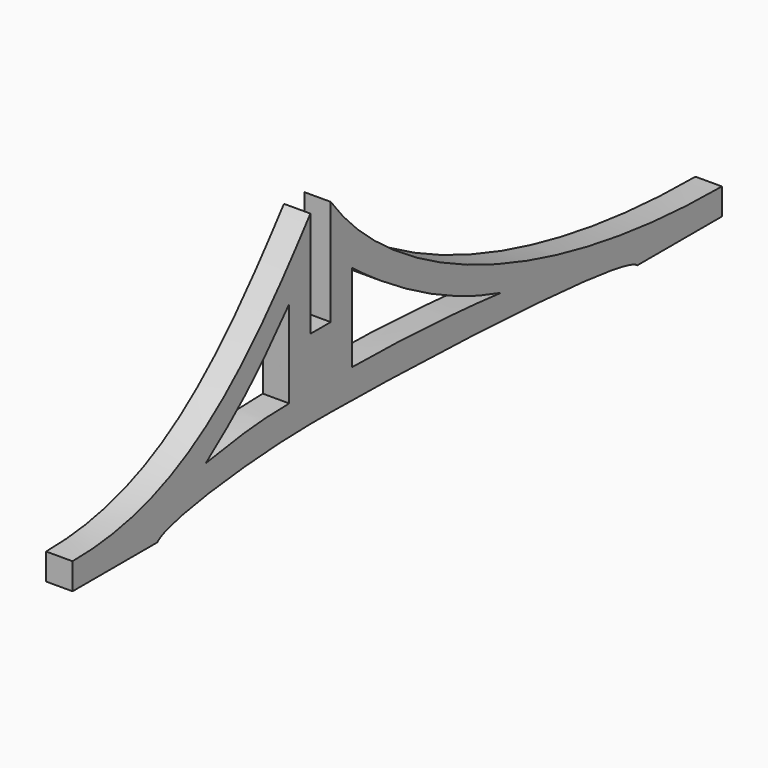
from build123d import *

# Parameters (mm, degrees)
F0_W     = 2.4
F0_H     = 15
F1_DEPTH = 5


# Not quite as in the source:
# - a feature names something its author has since deleted; it is built from what else it names


with BuildPart() as f1:
    # F0 (on Right) → F1 (new body)
    with BuildSketch(Plane.YZ):
        with Locations((-1.2, 12.5)):
            Rectangle(F0_W, F0_H)
        with Locations((1.2, 12.5)):
            Rectangle(F0_W, F0_H)
        with BuildLine():
            Line((2.4, 20), (2.4, 5))
            add(Edge.make_bspline(
                [(74.7971267972, 0), (71.3879865607, 3.4156564958), (16.494217181, 5), (2.4, 5)],
                knots=[0, 0, 0, 0, 72.5695801868, 72.5695801868, 72.5695801868, 72.5695801868], degree=3))
            Line((74.7971267972, 0), (94.7971267972, 0))
            Line((94.7971267972, 0), (94.7971267972, 5))
            add(Edge.make_bspline(
                [(2.4, 40), (16.6215170175, 20.5895993859), (51.1409416795, 5), (94.7971267972, 5)],
                knots=[0, 0, 0, 0, 98.8039930387, 98.8039930387, 98.8039930387, 98.8039930387], degree=3))
            Line((2.4, 40), (2.4, 20))
        make_face()
        with BuildLine():
            add(Edge.make_bspline(
                [(7.4, 27.0048175007), (7.4282917172, 21.6293986887), (7.3717082828, 15.8260287717), (7.4, 10.4506099597)],
                knots=[0, 0, 0, 0, 16.554207541, 16.554207541, 16.554207541, 16.554207541], degree=3))
            add(Edge.make_bspline(
                [(42.5923541188, 8.5242791101), (28.9157964289, 12.3093035072), (16.1028206348, 20.2473960817), (7.4, 27.0048175007)],
                knots=[0, 0, 0, 0, 39.7496174526, 39.7496174526, 39.7496174526, 39.7496174526], degree=3))
            add(Edge.make_bspline(
                [(7.4, 10.4506099597), (17.3497335032, 10.4361297563), (31.9942831993, 9.6850190312), (42.5923541188, 8.5242791101)],
                knots=[0, 0, 0, 0, 35.2450356641, 35.2450356641, 35.2450356641, 35.2450356641], degree=3))
        make_face(mode=Mode.SUBTRACT)
        with BuildLine():
            add(Edge.make_bspline(
                [(-2.4, 5), (-13.9117193222, 5), (-35.8368966605, 2.8542873915), (-38.5822232689, 0)],
                knots=[0, 0, 0, 0, 36.5260630329, 36.5260630329, 36.5260630329, 36.5260630329], degree=3))
            Line((-2.4, 5), (-2.4, 20))
            Line((-2.4, 20), (-2.4, 30.4898899049))
            Line((-2.4, 30.4898899049), (-2.4, 40))
            add(Edge.make_bspline(
                [(-58.5822232689, 5), (-32.4707888067, 5), (-18.0997792631, 19.8830608279), (-2.4, 40)],
                knots=[0, 0, 0, 0, 66.1924634036, 66.1924634036, 66.1924634036, 66.1924634036], degree=3))
            Line((-58.5822232689, 5), (-58.5822232689, 0))
            Line((-58.5822232689, 0), (-38.5822232689, 0))
        make_face()
        with BuildLine():
            add(Edge.make_bspline(
                [(-7.4, 27.0048175007), (-14.9471499026, 18.3299258351), (-18.6816509813, 14.8076107726), (-27.100559324, 8.5242791101)],
                knots=[0, 0, 0, 0, 27.0118925084, 27.0118925084, 27.0118925084, 27.0118925084], degree=3))
            add(Edge.make_bspline(
                [(-7.4, 27.0048175007), (-7.4600156685, 21.4867483204), (-7.3399843315, 15.96867914), (-7.4, 10.4506099597)],
                knots=[0, 0, 0, 0, 16.554207541, 16.554207541, 16.554207541, 16.554207541], degree=3))
            add(Edge.make_bspline(
                [(-27.100559324, 8.5242791101), (-19.2162878811, 9.7881155089), (-14.8515102789, 10.4084629565), (-7.4, 10.4506099597)],
                knots=[0, 0, 0, 0, 19.7945140941, 19.7945140941, 19.7945140941, 19.7945140941], degree=3))
        make_face(mode=Mode.SUBTRACT)
    extrude(amount=F1_DEPTH)


solid = f1.part
